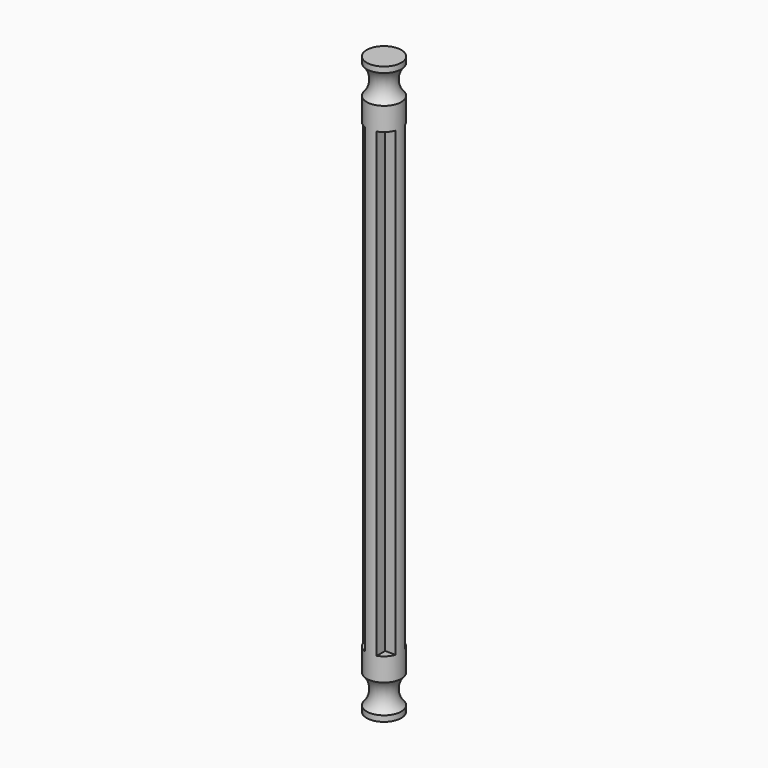
from build123d import *

# Parameters (mm, degrees)
F2_W          = 2
F2_H          = 2
F3_DEPTH      = 40
F3_DEPTH_BACK = 40


# Not quite as in the source:
# - a feature names something its author has since deleted; it is built from what else it names


with BuildPart() as f1:
    # F0 (on Front) → F1 (revolve)
    with BuildSketch(Plane.XZ):
        with BuildLine():
            Line((0, 50), (0, -50))
            Line((0, -50), (3, -50))
            Line((3, -50), (3, -49))
            ThreePointArc((3, -49), (2, -46.5), (3, -44))
            Line((3, -44), (3, 0))
            Line((3, 0), (3, 44))
            ThreePointArc((3, 44), (2, 46.5), (3, 49))
            Line((3, 49), (3, 50))
            Line((3, 50), (0, 50))
        make_face()
    revolve(axis=Axis((0, 0, 0), (0, 0, 1)))

    # F2 (on Top) → F3 (cut, two sides)
    with BuildSketch(Plane.XY) as f3_sk:
        with Locations((2, 2)):
            Rectangle(F2_W, F2_H)
        with Locations((-2, 2)):
            Rectangle(F2_W, F2_H)
        with Locations((-2, -2)):
            Rectangle(F2_W, F2_H)
        with Locations((2, -2)):
            Rectangle(F2_W, F2_H)
    extrude(amount=-F3_DEPTH, mode=Mode.SUBTRACT)
    extrude(f3_sk.sketch, amount=F3_DEPTH_BACK, mode=Mode.SUBTRACT)


solid = f1.part
